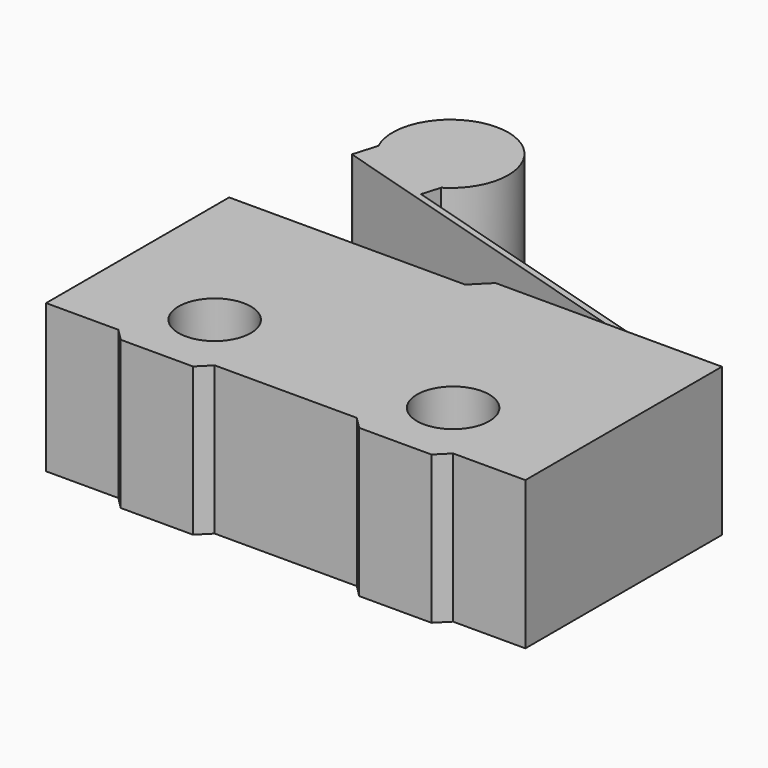
from build123d import *

# Parameters (mm, degrees)
F0_W          = 19.9
F0_H          = 10.7
F1_DEPTH      = 3.075
F1_DEPTH_BACK = 3.075
F2_W          = 1.5
F2_H          = 4
F3_DEPTH      = 1
F4_R          = 0.5
F6_DEPTH      = 4
F7_W          = 10.5
F7_H          = 0.7
F7_W_2        = 3.5
F7_H_2        = 0.5
F7_W_3        = 6.9
F7_R          = 1.5
F8_DEPTH      = 25
F9_SIZE       = 0.69999
F10_SIZE      = 0.49999


# Not quite as in the source:
# - a fillet or chamfer is up to 0.001 mm smaller than in the source, because OpenCascade refuses the exact size


with BuildPart() as f1:
    # F0 (on Top) → F1 (new body, two sides)
    with BuildSketch(Plane.XY) as f1_sk:
        Rectangle(F0_W, F0_H)
    extrude(amount=F1_DEPTH)
    extrude(f1_sk.sketch, amount=-F1_DEPTH_BACK)

    # F2 (on face) → F3 (join)
    with BuildSketch(Plane(origin=(0, 5.35, 0), x_dir=(-1, 0, 0), z_dir=(0, 1, 0))):
        with Locations((-3.2, 0)):
            Rectangle(F2_W, F2_H)
    extrude(amount=F3_DEPTH)

    # F4
    f4_edges = [f1.edges().sort_by_distance(p)[0] for p in [
        (2.45, 6.35, 0),
        (3.95, 6.35, 0),
    ]]
    fillet(f4_edges, radius=F4_R)

    # F5 (on face) → F6 (join)
    with BuildSketch(Plane(origin=(0, 0, -2), x_dir=(1, 0, 0), z_dir=(0, 0, -1))):
        with BuildLine():
            Line((6.75, -6.35), (6.75, -5.35))
            Line((6.75, -5.35), (6.5, -5.35))
            Line((6.5, -5.35), (6.5, -6.1638856134))
            Line((6.5, -6.1638856134), (-9.95, -11.089035314))
            Line((-9.95, -11.089035314), (-10.021705391, -11.110503994))
            Line((-10.021705391, -11.110503994), (-9.95, -11.35))
            Line((-9.95, -11.35), (-9.7212332774, -12.1140808536))
            ThreePointArc((-9.7212332774, -12.1140808536), (-6.8616282462, -15.4358597688), (-6.297976785, -11.08915376))
            Line((-6.297976785, -11.08915376), (-6.5267435076, -10.3250729065))
            Line((-6.5267435076, -10.3250729065), (6.75, -6.35))
        make_face()
    extrude(amount=-F6_DEPTH)

    # F7 (on face) → F8 (cut)
    with BuildSketch(Plane(origin=(0, 0, -3.075), x_dir=(1, 0, 0), z_dir=(0, 0, -1))):
        with Locations((-4.7, -5)):
            Rectangle(F7_W, F7_H)
        with Locations((-8.2, 5.1)):
            Rectangle(F7_W_2, F7_H_2)
        with Locations((8.2, 5.1)):
            Rectangle(F7_W_2, F7_H_2)
        with Locations((0, 5.1)):
            Rectangle(F7_W_3, F7_H_2)
        with Locations((4.95, 2.35)):
            Circle(F7_R)
        with Locations((-4.95, 2.35)):
            Circle(F7_R)
    extrude(amount=-F8_DEPTH, mode=Mode.SUBTRACT)

    # F9 (size 0.7 in the source; OpenCascade refuses exactly that, so slightly less here)
    f9_edges = [f1.edges().sort_by_distance(p)[0] for p in [
        (0.55, 4.65, 0),
    ]]
    chamfer(f9_edges, length=F9_SIZE)

    # F10 (size 0.5 in the source; OpenCascade refuses exactly that, so slightly less here)
    f10_edges = [f1.edges().sort_by_distance(p)[0] for p in [
        (6.45, -4.85, 0),
        (3.45, -4.85, 0),
        (-3.45, -4.85, 0),
        (-6.45, -4.85, 0),
    ]]
    chamfer(f10_edges, length=F10_SIZE)


solid = f1.part
